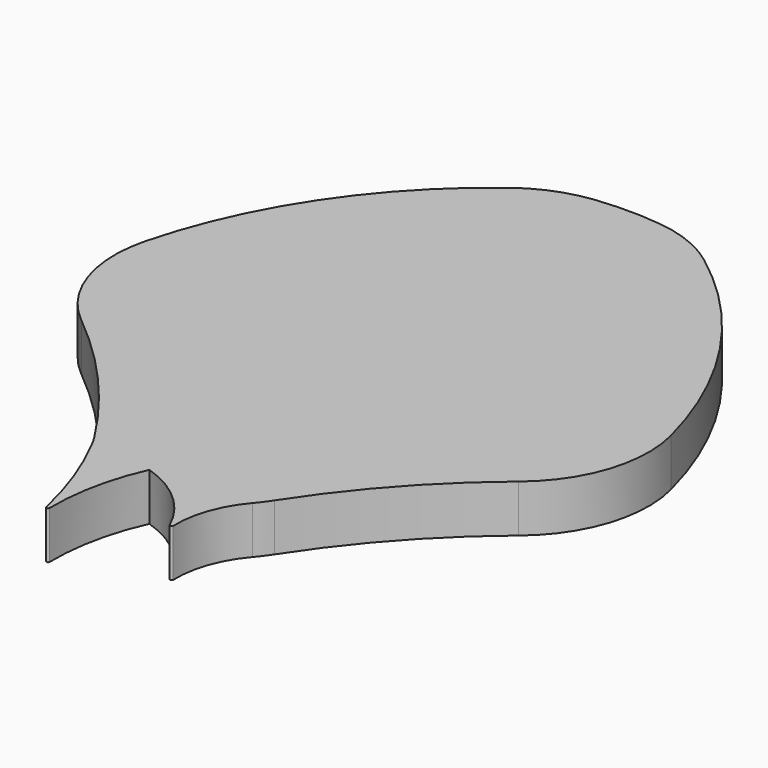
from build123d import *

# Parameters (mm, degrees)
F1_DEPTH    = 9
F2_DEPTH    = 9
F3_T1_DEPTH = 9
F3_T3_DEPTH = 97.7984007527
F3_T5_DEPTH = 18.7464853336
F3_T7_DEPTH = 44.8077335821
F4_F1_R     = 0.3
F4_F2_R     = 0.3


# Not quite as in the source:
# - a fillet or chamfer that OpenCascade refuses, or shapes differently, is made with other operations: its cross-section is extruded or revolved along the edge and cut away or added


with BuildPart() as f1:
    # F0 (on Top) → F1 (new body)
    with BuildSketch(Plane.XY):
        with BuildLine():
            ThreePointArc((52.3559108968, -15.2742949835), (41.1175441228, 23.5793695766), (13.2592789192, 52.9021456617))
            ThreePointArc((13.2592789192, 52.9021456617), (0, 54.5384771796), (-13.2592789192, 52.9021456617))
            ThreePointArc((-13.2592789192, 52.9021456617), (-41.1175441228, 23.5793695766), (-52.3559108968, -15.2742949835))
            ThreePointArc((-52.3559108968, -15.2742949835), (-32.1035122758, -31.703635387), (-15.9292943442, -52.1603592277))
            ThreePointArc((-15.9292943442, -52.1603592277), (-9.8139264878, -53.648227743), (-3.5678639787, -54.4216486309))
            ThreePointArc((-3.5678639787, -54.4216486309), (6.2832792085, -54.1753255224), (15.9292943442, -52.1603592277))
            ThreePointArc((15.9292943442, -52.1603592277), (32.1035122758, -31.703635387), (52.3559108968, -15.2742949835))
        make_face()
    extrude(amount=F1_DEPTH)

    # F0 (on Top) → F2 (join)
    with BuildSketch(Plane.XY):
        with BuildLine():
            ThreePointArc((-7.0224064402, -78.6131843925), (-7.0174520358, -66.2714702986), (-3.5678639787, -54.4216486309))
            ThreePointArc((-3.5678639787, -54.4216486309), (-9.8139264878, -53.648227743), (-15.9292943442, -52.1603592277))
            ThreePointArc((-15.9292943442, -52.1603592277), (-10.336712225, -65.0032144434), (-7.0224064402, -78.6131843925))
        make_face()
        with BuildLine():
            ThreePointArc((10.5660464615, -68.2554319501), (11.3560818324, -59.5775748336), (15.9292943442, -52.1603592277))
            ThreePointArc((15.9292943442, -52.1603592277), (6.2832792085, -54.1753255224), (-3.5678639787, -54.4216486309))
            ThreePointArc((-3.5678639787, -54.4216486309), (5.1525036315, -59.6492567371), (10.5660464615, -68.2554319501))
        make_face()
    extrude(amount=F2_DEPTH)

    # F3: fillet of radius 25 on 6 edges, made by hand

    # F3_s2 → F3_t1 (join)
    with BuildSketch(Plane.XY):
        with BuildLine():
            ThreePointArc((-16.4732265546, -51.2989033705), (-15.9263980679, -52.1979676734), (-15.4178890795, -53.1192475566))
            ThreePointArc((-15.4178890795, -53.1192475566), (-15.6719958304, -52.6389522584), (-15.9292943442, -52.1603592277))
            ThreePointArc((-15.9292943442, -52.1603592277), (-16.2003358533, -51.7290474995), (-16.4732265546, -51.2989033705))
        make_face()
    extrude(amount=F3_T1_DEPTH)

    # F3_s4 → F3_t3 (cut)
    with BuildSketch(Plane.XY.offset(-44.3992003763)):
        with BuildLine():
            ThreePointArc((41.3774463504, -23.2564339871), (49.2973579438, -11.704046911), (49.7610601076, 2.2947968664))
            ThreePointArc((49.7610601076, 2.2947968664), (51.5165033775, -6.4221025316), (52.3559108968, -15.2742949835))
            ThreePointArc((52.3559108968, -15.2742949835), (46.752445175, -19.108250225), (41.3774463504, -23.2564339871))
        make_face()
        with BuildLine():
            ThreePointArc((-49.7610601076, 2.2947968664), (-49.2973579438, -11.704046911), (-41.3774463504, -23.2564339871))
            ThreePointArc((-41.3774463504, -23.2564339871), (-46.752445175, -19.108250225), (-52.3559108968, -15.2742949835))
            ThreePointArc((-52.3559108968, -15.2742949835), (-51.5165033775, -6.4221025316), (-49.7610601076, 2.2947968664))
        make_face()
    extrude(amount=F3_T3_DEPTH, mode=Mode.SUBTRACT)

    # F3_s6 → F3_t5 (cut)
    with BuildSketch(Plane.XY.offset(-4.8732426668)):
        with BuildLine():
            ThreePointArc((16.9764615861, -50.5162181687), (16.0190019724, -51.8895795654), (14.9717711174, -53.195779387))
            ThreePointArc((14.9717711174, -53.195779387), (15.4409431776, -52.6692011973), (15.9292943442, -52.1603592277))
            ThreePointArc((15.9292943442, -52.1603592277), (16.4495016002, -51.3361382631), (16.9764615861, -50.5162181687))
        make_face()
    extrude(amount=F3_T5_DEPTH, mode=Mode.SUBTRACT)

    # F3_s8 → F3_t7 (cut)
    with BuildSketch(Plane.XY.offset(-17.903866791)):
        with BuildLine():
            ThreePointArc((18.4012083068, 49.3190772564), (12.6321038646, 52.5652026084), (6.2132770502, 54.1833985771))
            ThreePointArc((6.2132770502, 54.1833985771), (9.7573311543, 53.6585499414), (13.2592789192, 52.9021456617))
            ThreePointArc((13.2592789192, 52.9021456617), (15.8631283238, 51.1578030954), (18.4012083068, 49.3190772564))
        make_face()
        with BuildLine():
            ThreePointArc((-6.2132770502, 54.1833985771), (-12.6321038646, 52.5652026084), (-18.4012083068, 49.3190772564))
            ThreePointArc((-18.4012083068, 49.3190772564), (-15.8631283238, 51.1578030954), (-13.2592789192, 52.9021456617))
            ThreePointArc((-13.2592789192, 52.9021456617), (-9.7573311543, 53.6585499414), (-6.2132770502, 54.1833985771))
        make_face()
    extrude(amount=F3_T7_DEPTH, mode=Mode.SUBTRACT)

    # F4: fillet of radius 0.3 on 2 edges, made by hand

    # F4_f1
    f4_f1_edges = [f1.edges().sort_by_distance(p)[0] for p in [
        (-7.0224064402, -78.6131843925, 4.5),
    ]]
    fillet(f4_f1_edges, radius=F4_F1_R)

    # F4_f2
    f4_f2_edges = [f1.edges().sort_by_distance(p)[0] for p in [
        (10.5660464615, -68.2554319501, 4.5),
    ]]
    fillet(f4_f2_edges, radius=F4_F2_R)


solid = f1.part
